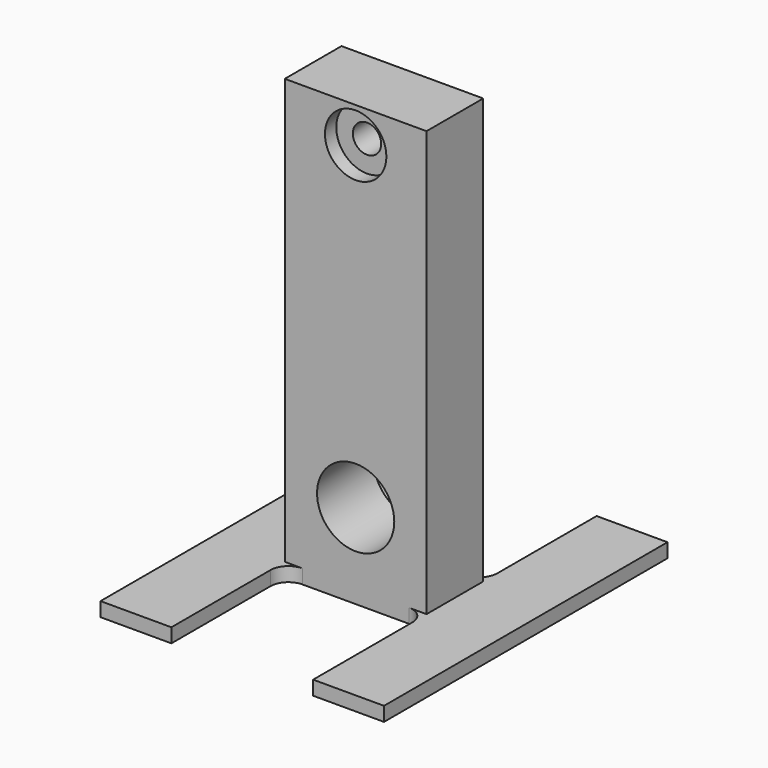
from build123d import *

# Parameters (mm, degrees)
F0_W      = 25.4
F0_H      = 127
F1_DEPTH  = 25.4
F2_W      = 50.8
F2_H      = 25.4
F3_DEPTH  = 25.4
F4_R      = 5.08
F5_DEPTH  = 25.4
F6_R      = 11.0109
F7_DEPTH  = 5.08
F8_R      = 11.0109
F9_DEPTH  = 5.08
F10_DEPTH = 25.4
F11_W     = 25.4
F11_H     = 127
F12_DEPTH = 12.7
F13_DEPTH = 12.7
F14_R     = 13.83665
F15_DEPTH = 25.4
F17_DEPTH = 5.08


with BuildPart() as f1:
    # F0 (on Front) → F1 (new body)
    with BuildSketch(Plane.XZ):
        with Locations((-12.3247115396, -29.6700978652)):
            Rectangle(F0_W, F0_H)
    extrude(amount=F1_DEPTH)

    # F2 (on face) → F3 (join)
    with BuildSketch(Plane.XY.offset(33.8299021348)):
        with Locations((-12.3247115396, -12.7)):
            Rectangle(F2_W, F2_H)
    extrude(amount=F3_DEPTH)

    # F4 (on face) → F5 (cut)
    with BuildSketch(Plane.XZ.offset(25.4)):
        with Locations((-12.3247115396, 46.5299021348)):
            Circle(F4_R)
    extrude(amount=-F5_DEPTH, mode=Mode.SUBTRACT)

    # F6 (on face) → F7 (cut)
    with BuildSketch(Plane.XZ.offset(25.4)):
        with Locations((-12.3247115396, 46.5299021348)):
            Circle(F6_R)
    extrude(amount=-F7_DEPTH, mode=Mode.SUBTRACT)

    # F8 (on face) → F9 (cut)
    with BuildSketch(Plane(origin=(0, 0, 0), x_dir=(-1, 0, 0), z_dir=(0, 1, 0))):
        with Locations((12.3247115396, 46.5299021348)):
            Circle(F8_R)
    extrude(amount=-F9_DEPTH, mode=Mode.SUBTRACT)

    # F4 (on face) → F10 (cut)
    with BuildSketch(Plane.XZ.offset(25.4)):
        with Locations((-12.3247115396, 46.5299021348)):
            Circle(F4_R)
    extrude(amount=-F10_DEPTH, mode=Mode.SUBTRACT)

    # F11 (on face) → F12 (join)
    with BuildSketch(Plane(origin=(-25.0247115396, 0, 0), x_dir=(0, -1, 0), z_dir=(-1, 0, 0))):
        with Locations((12.7, -29.6700978652)):
            Rectangle(F11_W, F11_H)
    extrude(amount=F12_DEPTH)

    # F13 (add): a face of the model
    f13_faces = [f1.faces().sort_by_distance(p)[0] for p in [
        (0.3752884604, -12.7, -29.6700978652),
    ]]
    extrude(f13_faces, amount=F13_DEPTH)

    # F14 (on face) → F15 (cut)
    with BuildSketch(Plane.XZ.offset(25.4)):
        with Locations((-12.3247115396, -67.7700978652)):
            Circle(F14_R)
    extrude(amount=-F15_DEPTH, mode=Mode.SUBTRACT)

    # F16 (on face) → F17 (join)
    with BuildSketch(Plane(origin=(0, 0, -93.1700978652), x_dir=(1, 0, 0), z_dir=(0, 0, -1))):
        with BuildLine():
            ThreePointArc((-37.7247115396, -6.35), (-35.8648396001, -1.8598719395), (-31.3747115396, 0))
            Line((-31.3747115396, 0), (6.7252884604, 0))
            ThreePointArc((6.7252884604, 0), (11.2154165209, -1.8598719395), (13.0752884604, -6.35))
            Line((13.0752884604, -6.35), (13.0752884604, -50.8))
            Line((13.0752884604, -50.8), (38.4752884604, -50.8))
            Line((38.4752884604, -50.8), (38.4752884604, 0))
            Line((38.4752884604, 0), (38.4752884604, 25.4))
            Line((38.4752884604, 25.4), (38.4752884604, 76.2))
            Line((38.4752884604, 76.2), (13.0752884604, 76.2))
            Line((13.0752884604, 76.2), (13.0752884604, 31.75))
            ThreePointArc((13.0752884604, 31.75), (11.2154165209, 27.2598719395), (6.7252884604, 25.4))
            Line((6.7252884604, 25.4), (-31.3747115396, 25.4))
            ThreePointArc((-31.3747115396, 25.4), (-35.8648396001, 27.2598719395), (-37.7247115396, 31.75))
            Line((-37.7247115396, 31.75), (-37.7247115396, 76.2))
            Line((-37.7247115396, 76.2), (-63.1247115396, 76.2))
            Line((-63.1247115396, 76.2), (-63.1247115396, 25.4))
            Line((-63.1247115396, 25.4), (-63.1247115396, 0))
            Line((-63.1247115396, 0), (-63.1247115396, -50.8))
            Line((-63.1247115396, -50.8), (-37.7247115396, -50.8))
            Line((-37.7247115396, -50.8), (-37.7247115396, -6.35))
        make_face()
    extrude(amount=F17_DEPTH)


solid = f1.part
